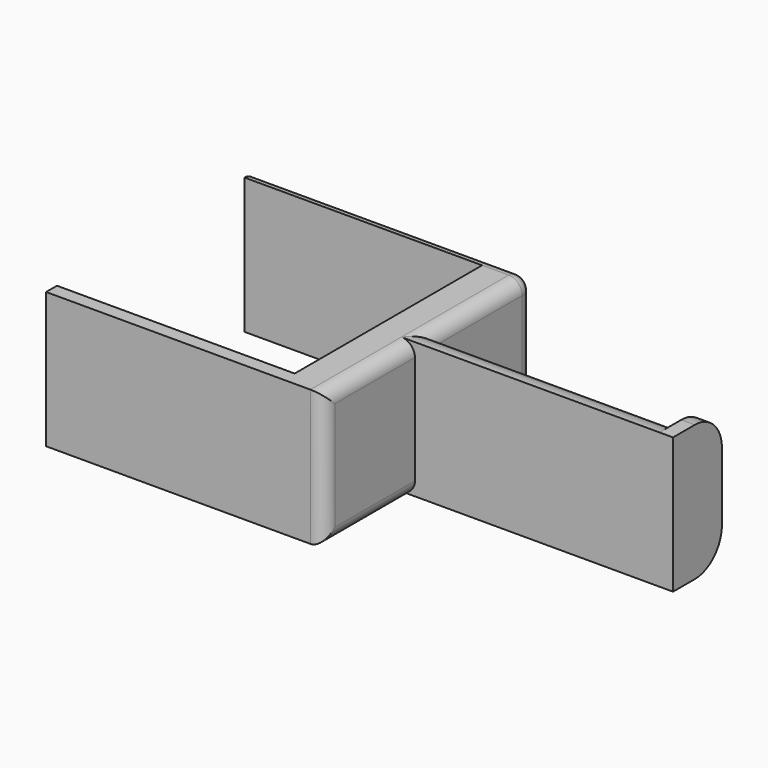
from build123d import *

# Parameters (mm, degrees)
F0_W         = 35
F0_H         = 2
F0_W_2       = 2
F0_H_2       = 4
F1_DEPTH     = 20
F2_R         = 4.99999
F3_R         = 5
F4_R         = 2
F5_T1_DEPTH  = 43.9093010689
F5_S5_W      = 2
F5_S5_H      = 2
F5_T6_DEPTH  = 2
F5_S11_W     = 2
F5_S11_H     = 2
F5_T12_DEPTH = 2


# Not quite as in the source:
# - a fillet or chamfer that OpenCascade refuses, or shapes differently, is made with other operations: its cross-section is extruded or revolved along the edge and cut away or added
# - a fillet or chamfer is up to 0.001 mm smaller than in the source, because OpenCascade refuses the exact size


with BuildPart() as f1:
    # F0 (on Top) → F1 (new body)
    with BuildSketch(Plane.XY):
        with Locations((-20.4546505344, 18.25)):
            Rectangle(F0_W, F0_H)
        Polygon((2.9546505344, 2.5), (2.9546505344, 19.25), (-2.9546505344, 19.25), (-2.9546505344, 17.25), (-2.9546505344, -17.25), (-2.9546505344, -19.25), (2.9546505344, -19.25), (2.9546505344, -2.5), align=None)
        Polygon((38.9546505344, 2.5), (2.9546505344, 2.5), (2.9546505344, -2.5), (40.9546505344, -2.5), (40.9546505344, 2.5), align=None)
        with Locations((39.9546505344, 4.5)):
            Rectangle(F0_W_2, F0_H_2)
        with Locations((-20.4546505344, -18.25)):
            Rectangle(F0_W, F0_H)
    extrude(amount=F1_DEPTH)

    # F2 (radius 5 in the source; OpenCascade refuses exactly that, so slightly less here)
    f2_edges = [f1.edges().sort_by_distance(p)[0] for p in [
        (20.954651, 2.5, 20),
        (20.954651, 2.5, 0),
    ]]
    fillet(f2_edges, radius=F2_R)

    # F3
    f3_edges = [f1.edges().sort_by_distance(p)[0] for p in [
        (39.954651, 6.5, 20),
        (39.954651, 6.5, 0),
    ]]
    fillet(f3_edges, radius=F3_R)

    # F4
    f4_edges = [f1.edges().sort_by_distance(p)[0] for p in [
        (2.954651, 10.875, 20),
        (2.954651, -10.875, 20),
        (2.954651, 10.875, 0),
        (2.954651, -10.875, 0),
        (2.954651, 19.25, 10),
        (2.954651, -19.25, 10),
    ]]
    fillet(f4_edges, radius=F4_R)

    # F5: fillet of radius 2 on 2 edges, made by hand

    # F5_s2 → F5_t1 (cut)
    with BuildSketch(Plane.YZ.offset(-42.9546505344)):
        with BuildLine():
            ThreePointArc((17.25, 0), (18.6642135624, 0.5857864376), (19.25, 2))
            Line((19.25, 2), (19.25, 0))
            Line((19.25, 0), (17.25, 0))
        make_face()
        with BuildLine():
            ThreePointArc((19.25, 18), (18.6642135624, 19.4142135624), (17.25, 20))
            Line((17.25, 20), (19.25, 20))
            Line((19.25, 20), (19.25, 18))
        make_face()
    extrude(amount=F5_T1_DEPTH, mode=Mode.SUBTRACT)


with BuildPart() as f5_tool4:
    # F5_s5 → F5_t6 (new body)
    with BuildSketch(Plane.XZ.offset(-17.25)):
        with Locations((1.9546505344, 19)):
            Rectangle(F5_S5_W, F5_S5_H)
    extrude(amount=-F5_T6_DEPTH)

    # F5_s7 → F5_t8 (revolve, cut)
    with BuildSketch(Plane(origin=(0.9546505344, 17.25, 18), x_dir=(-0.7071067812, 0, -0.7071067812), z_dir=(0.7071067812, 0, -0.7071067812))):
        with BuildLine():
            ThreePointArc((0, -2), (2, 0), (0, 2))
            Line((0, 2), (0, -2))
        make_face()
    revolve(axis=Axis((0.9546505344, 17.25, 18), (0, 1, 0)), mode=Mode.SUBTRACT)


with BuildPart() as f1_1:
    add(f1.part)

    # F5_t3: cut F5_tool4
    add(f5_tool4.part, mode=Mode.SUBTRACT)


with BuildPart() as f5_tool10:
    # F5_s11 → F5_t12 (new body)
    with BuildSketch(Plane.XY.offset(2)):
        with Locations((1.9546505344, 18.25)):
            Rectangle(F5_S11_W, F5_S11_H)
    extrude(amount=-F5_T12_DEPTH)

    # F5_s13 → F5_t14 (revolve, cut)
    with BuildSketch(Plane(origin=(0.9546505344, 17.25, 2), x_dir=(-0.7071067812, -0.7071067812, 0), z_dir=(0.7071067812, -0.7071067812, 0))):
        with BuildLine():
            ThreePointArc((0, -2), (2, 0), (0, 2))
            Line((0, 2), (0, -2))
        make_face()
    revolve(axis=Axis((0.9546505344, 17.25, 2), (0, 0, -1)), mode=Mode.SUBTRACT)


with BuildPart() as f1_2:
    add(f1_1.part)

    # F5_t9: cut F5_tool10
    add(f5_tool10.part, mode=Mode.SUBTRACT)


solid = f1_2.part
